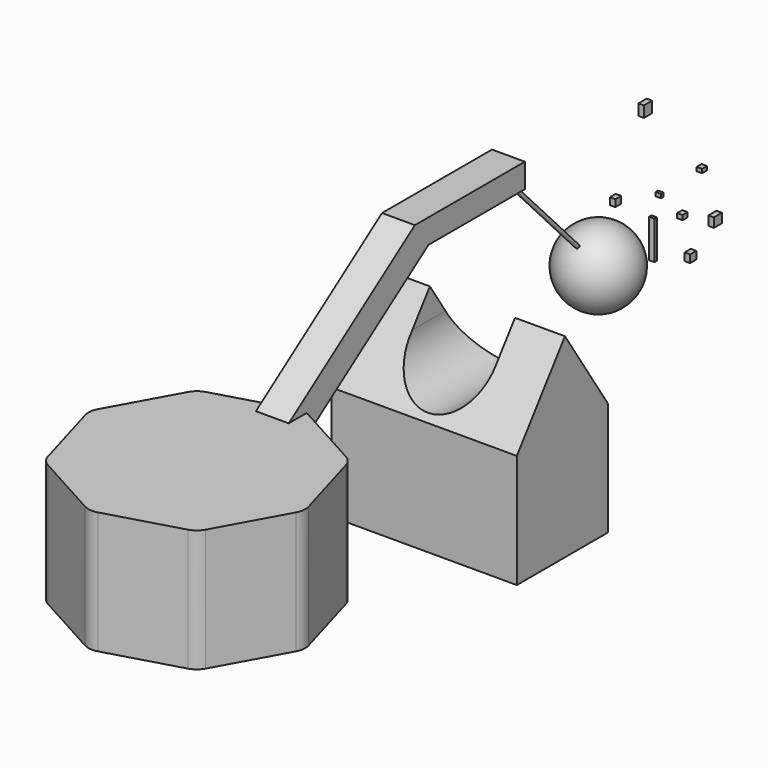
from build123d import *

# Parameters (mm, degrees)
F1_DEPTH      = 67.818
F4_W          = 18.2206444442
F4_H          = 16.4148422464
F5_DEPTH      = 35.052
F5_DEPTH_BACK = 81.28
F7_W          = 18.2206444442
F7_H          = 13.4462515828
F8_DEPTH      = 76.2
F12_DEPTH     = 51.308
F14_DEPTH     = 307.34
F15_W         = 3.5439252173
F15_H         = 2.5313720107
F16_DEPTH     = 3.048
F15_W_2       = 5.5693387985
F15_H_2       = 5.1409378648
F15_W_3       = 4.2840838432
F15_H_3       = 4.2841136456
F15_W_4       = 1.7136335373
F15_H_4       = 2.1420568228
F15_W_5       = 1.678943634
F15_H_5       = 21.2063714862
F15_W_6       = 4.0373813916
F15_H_6       = 3.8556978106
F15_W_7       = 3.4273266792
F15_W_8       = 5.7214427742
F15_H_7       = 6.1301365495


with BuildPart() as f1:
    # F0 (on Top) → F1 (new body)
    with BuildSketch(Plane.XY):
        with BuildLine():
            Line((-3.3124033153, -64.5529893688), (37.227621348, -52.8409373586))
            ThreePointArc((37.227621348, -52.8409373586), (40.7482742502, -51.0188053655), (43.3036336822, -47.9880793748))
            Line((43.3036336822, -47.9880793748), (63.6880886331, -11.0402816279))
            ThreePointArc((63.6880886331, -11.0402816279), (64.8891242859, -7.262362198), (64.5529893688, -3.3124033153))
            Line((64.5529893688, -3.3124033153), (52.8409373586, 37.227621348))
            ThreePointArc((52.8409373586, 37.227621348), (51.0188053655, 40.7482742502), (47.9880793748, 43.3036336822))
            Line((47.9880793748, 43.3036336822), (11.0402816279, 63.6880886331))
            ThreePointArc((11.0402816279, 63.6880886331), (7.262362198, 64.8891242859), (3.3124033153, 64.5529893688))
            Line((3.3124033153, 64.5529893688), (-37.227621348, 52.8409373586))
            ThreePointArc((-37.227621348, 52.8409373586), (-40.7482742502, 51.0188053655), (-43.3036336822, 47.9880793748))
            Line((-43.3036336822, 47.9880793748), (-63.6880886331, 11.0402816279))
            ThreePointArc((-63.6880886331, 11.0402816279), (-64.8891242859, 7.262362198), (-64.5529893688, 3.3124033153))
            Line((-64.5529893688, 3.3124033153), (-52.8409373586, -37.227621348))
            ThreePointArc((-52.8409373586, -37.227621348), (-51.0188053655, -40.7482742502), (-47.9880793748, -43.3036336822))
            Line((-47.9880793748, -43.3036336822), (-11.0402816279, -63.6880886331))
            ThreePointArc((-11.0402816279, -63.6880886331), (-7.262362198, -64.8891242859), (-3.3124033153, -64.5529893688))
        make_face()
    extrude(amount=F1_DEPTH)

    # F4 (on line) → F5 (join, two sides)
    with BuildSketch(Plane(origin=(0, 87.7434991713, 61.4386595487), x_dir=(1, 0, 0), z_dir=(0, -0.8191520443, -0.5735764364))) as f5_sk:
        with Locations((0, 17.3605981536)):
            Rectangle(F4_W, F4_H)
    extrude(amount=F5_DEPTH)
    extrude(f5_sk.sketch, amount=-F5_DEPTH_BACK)

    # F7 (on plane+point) → F8 (join)
    with BuildSketch(Plane.XZ.offset(-139.6589639498)):
        with Locations((0, 122.2799217629)):
            Rectangle(F7_W, F7_H)
    extrude(amount=-F8_DEPTH)


with BuildPart() as f10:
    # F9 (on Right) → F10 (revolve)
    with BuildSketch(Plane.YZ):
        with BuildLine():
            Line((213.895842433, 116.4420843124), (262.8673623017, 64.581070459))
            ThreePointArc((262.8673623017, 64.581070459), (263.0859847021, 35.038088053), (292.6256896875, 34.5467281301))
            Line((292.6256896875, 34.5467281301), (278.1074935259, 49.9215495422))
            Line((278.1074935259, 49.9215495422), (214.6345443587, 117.1396286399))
            Line((214.6345443587, 117.1396286399), (213.895842433, 116.4420843124))
        make_face()
    revolve(axis=Axis((0, 246.3710189423, 83.5305890911), (0, 0.6865618304, -0.7270714222)))


with BuildPart() as f12:
    # F11 (on Right) → F12 (new body, symmetric)
    with BuildSketch(Plane.YZ):
        Polygon((157.5710592777, -40.2006159251), (220.6147791832, -40.2006159251), (220.6147791832, 22.8431193803), (190.8941715956, 67.6941946149), (157.5710592777, 22.8431193803), align=None)
    extrude(amount=F12_DEPTH, both=True)

    # F13 (on Front) → F14 (cut)
    with BuildSketch(Plane.XZ):
        with BuildLine():
            Line((-23.5774199521, 92.2675209238), (-23.5774199521, 51.3375234856))
            ThreePointArc((-23.5774199521, 51.3375234856), (-0.4440142616, 26.1994476979), (23.6177416804, 50.4504108568))
            Line((23.6177416804, 50.4504108568), (23.6177416804, 86.8789901563))
            Line((23.6177416804, 86.8789901563), (-23.5774199521, 92.2675209238))
        make_face()
    extrude(amount=-F14_DEPTH, mode=Mode.SUBTRACT)


with BuildPart() as f16:
    # F15 (on Right) → F16 (new body)
    with BuildSketch(Plane.YZ):
        with Locations((334.5247149807, 52.1797649562)):
            Rectangle(F15_W, F15_H)
    extrude(amount=F16_DEPTH)


with BuildPart() as f16b:
    # F15 (on Right) → F16, piece 2 (new body)
    with BuildSketch(Plane.YZ):
        with Locations((357.2113215923, 40.9406758845)):
            Rectangle(F15_W_2, F15_H_2)
    extrude(amount=F16_DEPTH)


with BuildPart() as f16c:
    # F15 (on Right) → F16, piece 3 (new body)
    with BuildSketch(Plane.YZ):
        with Locations((340.0748670101, 30.0161801279)):
            Rectangle(F15_W_3, F15_H_3)
    extrude(amount=F16_DEPTH)


with BuildPart() as f16d:
    # F15 (on Right) → F16, piece 4 (new body)
    with BuildSketch(Plane.YZ):
        with Locations((318.6542987823, 68.7874257565)):
            Rectangle(F15_W_4, F15_H_4)
    extrude(amount=F16_DEPTH)


with BuildPart() as f16e:
    # F15 (on Right) → F16, piece 5 (new body)
    with BuildSketch(Plane.YZ):
        with Locations((314.1385912895, 48.9733926952)):
            Rectangle(F15_W_5, F15_H_5)
    extrude(amount=F16_DEPTH)


with BuildPart() as f16f:
    # F15 (on Right) → F16, piece 6 (new body)
    with BuildSketch(Plane.YZ):
        with Locations((288.1462270116, 78.2124809921)):
            Rectangle(F15_W_6, F15_H_6)
    extrude(amount=F16_DEPTH)


with BuildPart() as f16g:
    # F15 (on Right) → F16, piece 7 (new body)
    with BuildSketch(Plane.YZ):
        with Locations((348.0004966259, 69.4300457835)):
            Rectangle(F15_W_7, F15_H_4)
    extrude(amount=F16_DEPTH)


with BuildPart() as f16h:
    # F15 (on Right) → F16, piece 8 (new body)
    with BuildSketch(Plane.YZ):
        with Locations((308.8307416065, 114.8136593401)):
            Rectangle(F15_W_8, F15_H_7)
    extrude(amount=F16_DEPTH)


solid = Compound([f1.part, f10.part, f12.part, f16.part, f16b.part, f16c.part, f16d.part, f16e.part, f16f.part, f16g.part, f16h.part])
